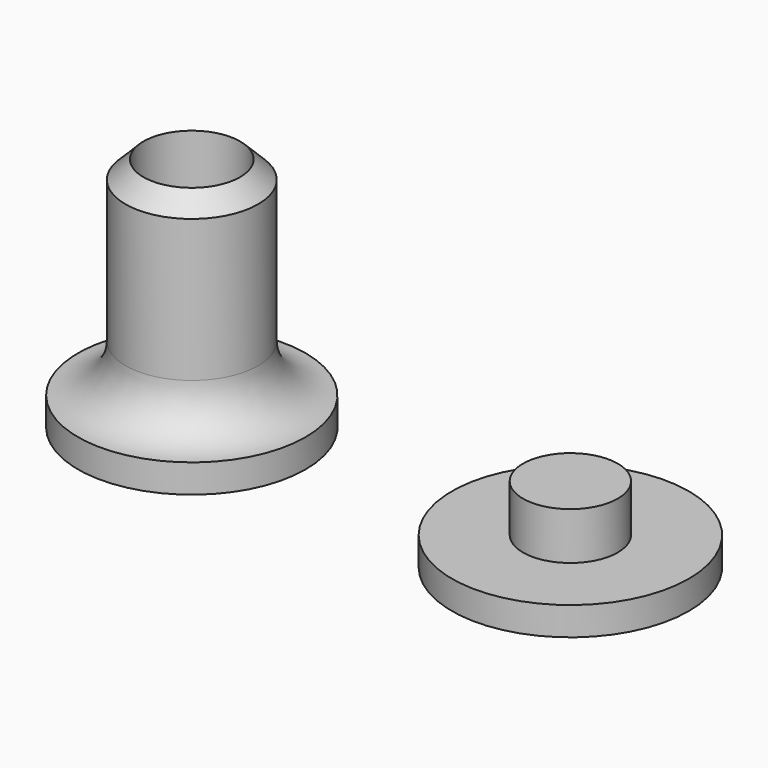
from build123d import *

# Parameters (mm, degrees)
F0_R     = 7
F0_R_2   = 5.1
F1_DEPTH = 25
F0_R_3   = 12
F2_DEPTH = 3
F3_R     = 4.99999
F5_R     = 12.5
F6_DEPTH = 3
F7_R     = 5
F8_DEPTH = 5


# Not quite as in the source:
# - a fillet or chamfer that OpenCascade refuses, or shapes differently, is made with other operations: its cross-section is extruded or revolved along the edge and cut away or added
# - a fillet or chamfer is up to 0.001 mm smaller than in the source, because OpenCascade refuses the exact size


with BuildPart() as f1:
    # F0 (on Top) → F1 (new body)
    with BuildSketch(Plane.XY):
        Circle(F0_R)
        Circle(F0_R_2, mode=Mode.SUBTRACT)
    extrude(amount=F1_DEPTH)

    # F0 (on Top) → F2 (join)
    with BuildSketch(Plane.XY):
        Circle(F0_R_3)
        Circle(F0_R, mode=Mode.SUBTRACT)
    extrude(amount=F2_DEPTH)

    # F3 (radius 5 in the source; OpenCascade refuses exactly that, so slightly less here)
    f3_edges = [f1.edges().sort_by_distance(p)[0] for p in [
        (-7, 0, 3),
    ]]
    fillet(f3_edges, radius=F3_R)

    # F4: chamfer of 2 on 1 edges, made by hand

    # F4_s1 → F4_t2 (revolve, cut)
    with BuildSketch(Plane.XZ):
        Polygon((7, 23), (5, 25), (7, 25), align=None)
    revolve(axis=Axis((0, 0, 25), (0, 0, 1)), mode=Mode.SUBTRACT)


with BuildPart() as f6:
    # F5 (on Top) → F6 (new body)
    with BuildSketch(Plane.XY):
        with Locations((39.9270130853, 0)):
            Circle(F5_R)
    extrude(amount=F6_DEPTH)

    # F7 (on face) → F8 (join)
    with BuildSketch(Plane.XY.offset(3)):
        with Locations((39.9270130853, 0)):
            Circle(F7_R)
    extrude(amount=F8_DEPTH)


solid = Compound([f1.part, f6.part])
